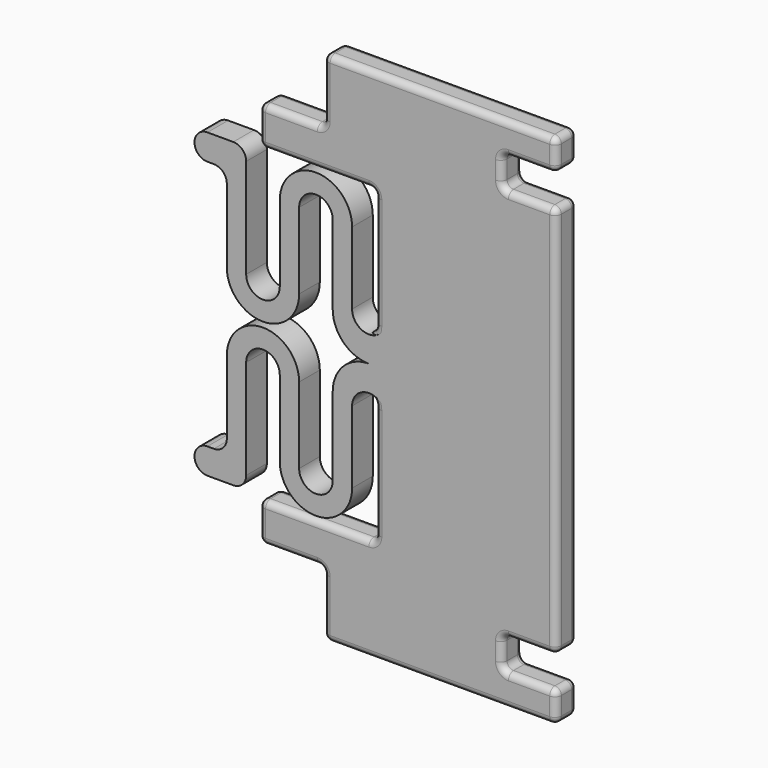
from build123d import *

# Parameters (mm, degrees)
F0_W          = 18
F0_H          = 2
F1_DEPTH      = 20
F2_W          = 4.2
F2_H          = 2.4
F3_DEPTH      = 2.001
F4_W          = 4
F4_H          = 12
F5_DEPTH      = 2.001
F6_W          = 5
F6_H          = 3
F7_DEPTH      = 2
F8_T1_DEPTH   = 2
F8_T3_DEPTH   = 2
F8_T5_DEPTH   = 7
F8_T7_DEPTH   = 7
F8_T9_DEPTH   = 7
F9_T1_DEPTH   = 2
F9_T3_DEPTH   = 18.75
F9_T5_DEPTH   = 1
F9_T7_DEPTH   = 4.5
F9_T9_DEPTH   = 3.15
F9_T11_DEPTH  = 17.7
F9_T13_DEPTH  = 5.5
F9_S17_W      = 0.5
F9_S17_H      = 0.5
F9_T18_DEPTH  = 0.5
F9_S23_W      = 0.5
F9_S23_H      = 0.5
F9_T24_DEPTH  = 0.5
F9_T27_DEPTH  = 1.4
F9_T29_DEPTH  = 3.2
F9_T31_DEPTH  = 8
F9_T33_DEPTH  = 4
F9_T35_DEPTH  = 4
F9_T37_DEPTH  = 8.6339745962
F9_S41_W      = 0.5
F9_S41_H      = 0.5
F9_T42_DEPTH  = 0.5
F9_S47_W      = 0.5
F9_S47_H      = 0.5
F9_T48_DEPTH  = 0.5
F9_S53_W      = 0.5
F9_S53_H      = 0.5
F9_T54_DEPTH  = 0.5
F9_S59_W      = 0.5
F9_S59_H      = 0.5
F9_T60_DEPTH  = 0.5
F9_S65_W      = 0.5
F9_S65_H      = 0.5
F9_T66_DEPTH  = 0.5
F9_S71_W      = 0.5
F9_S71_H      = 0.5
F9_T72_DEPTH  = 0.5
F9_S77_W      = 0.5
F9_S77_H      = 0.5
F9_T78_DEPTH  = 0.5
F9_S83_W      = 0.5
F9_S83_H      = 0.5
F9_T84_DEPTH  = 0.5
F9_S89_W      = 0.5
F9_S89_H      = 0.5
F9_T90_DEPTH  = 0.5
F9_S95_W      = 0.5
F9_S95_H      = 0.5
F9_T96_DEPTH  = 0.5
F9_T102_ANGLE = 131.6325091679
F9_S103_R     = 1.3
F9_T104_DEPTH = 3
F9_T108_ANGLE = 131.6325091679
F9_S109_R     = 1.3
F9_T110_DEPTH = 3
F9_T112_ANGLE = 90
F9_T114_ANGLE = 90
F9_T116_ANGLE = 90
F9_T118_ANGLE = 90
F9_T120_ANGLE = 90
F9_T122_ANGLE = 90
F9_T124_ANGLE = 90
F9_T126_ANGLE = 90


# Not quite as in the source:
# - a fillet or chamfer that OpenCascade refuses, or shapes differently, is made with other operations: its cross-section is extruded or revolved along the edge and cut away or added


with BuildPart() as f1:
    # F0 (on Top) → F1 (new body)
    with BuildSketch(Plane.XY):
        with Locations((-9, 1)):
            Rectangle(F0_W, F0_H)
    extrude(amount=F1_DEPTH)

    # F2 (on Front) → F3 (cut, through all)
    with BuildSketch(Plane.XZ):
        with Locations((-2.1, 16.4)):
            Rectangle(F2_W, F2_H)
    extrude(amount=-F3_DEPTH, mode=Mode.SUBTRACT)

    # F4 (on Front) → F5 (cut, through all)
    with BuildSketch(Plane.XZ):
        with Locations((-16, 6)):
            Rectangle(F4_W, F4_H)
    extrude(amount=-F5_DEPTH, mode=Mode.SUBTRACT)

    # F6 (on Front) → F7 (join)
    with BuildSketch(Plane.XZ):
        with BuildLine():
            Line((-24, 3), (-24, 11.7))
            Line((-24, 11.7), (-28, 11.7))
            Line((-28, 11.7), (-28, 9.7))
            Line((-28, 9.7), (-25.5, 9.7))
            Line((-25.5, 9.7), (-25.5, 3))
            ThreePointArc((-25.5, 3), (-22.7, 0.2), (-19.9, 3))
            Line((-19.9, 3), (-19.9, 8.9))
            ThreePointArc((-19.9, 8.9), (-18.6, 10.2), (-17.3, 8.9))
            Line((-17.3, 8.9), (-17.3, 2.8))
            ThreePointArc((-17.3, 2.8), (-16.4798989873, 0.8201010127), (-14.5, 0))
            Line((-14.5, 0), (-14, 0))
            Line((-14, 0), (-14, 2))
            Line((-14, 2), (-14.5, 2))
            ThreePointArc((-14.5, 2), (-15.4192388155, 2.3807611845), (-15.8, 3.3))
            Line((-15.8, 3.3), (-15.8, 8.9))
            ThreePointArc((-15.8, 8.9), (-18.6, 11.7), (-21.4, 8.9))
            Line((-21.4, 8.9), (-21.4, 3))
            ThreePointArc((-21.4, 3), (-22.7, 1.7), (-24, 3))
        make_face()
        with Locations((-20.5, 13.5)):
            Rectangle(F6_W, F6_H)
    extrude(amount=-F7_DEPTH)

    # F8: fillet of radius 1 on 5 edges, made by hand

    # F8_s2 → F8_t1 (join)
    with BuildSketch(Plane.XZ.offset(-2)):
        with BuildLine():
            ThreePointArc((-14, 2.8660254038), (-14.1339745962, 2.3660254038), (-14.5, 2))
            Line((-14.5, 2), (-14, 2))
            Line((-14, 2), (-14, 2.8660254038))
        make_face()
    extrude(amount=F8_T1_DEPTH)

    # F8_s4 → F8_t3 (join)
    with BuildSketch(Plane.XZ.offset(-2)):
        with BuildLine():
            ThreePointArc((-25.5, 8.7), (-25.7928932188, 9.4071067812), (-26.5, 9.7))
            Line((-26.5, 9.7), (-25.5, 9.7))
            Line((-25.5, 9.7), (-25.5, 8.7))
        make_face()
    extrude(amount=F8_T3_DEPTH)

    # F8_s6 → F8_t5 (cut)
    with BuildSketch(Plane.XZ.offset(-4.5)):
        with BuildLine():
            ThreePointArc((-25, 11.7), (-24.2928932188, 11.4071067812), (-24, 10.7))
            Line((-24, 10.7), (-24, 11.7))
            Line((-24, 11.7), (-25, 11.7))
        make_face()
    extrude(amount=F8_T5_DEPTH, mode=Mode.SUBTRACT)

    # F8_s8 → F8_t7 (cut)
    with BuildSketch(Plane.XZ.offset(-4.5)):
        with BuildLine():
            ThreePointArc((-27, 11.7), (-27.7071067812, 11.4071067812), (-28, 10.7))
            Line((-28, 10.7), (-28, 11.7))
            Line((-28, 11.7), (-27, 11.7))
        make_face()
    extrude(amount=F8_T7_DEPTH, mode=Mode.SUBTRACT)

    # F8_s10 → F8_t9 (cut)
    with BuildSketch(Plane.XZ.offset(-4.5)):
        with BuildLine():
            ThreePointArc((-28, 10.7), (-27.7071067812, 9.9928932188), (-27, 9.7))
            Line((-27, 9.7), (-28, 9.7))
            Line((-28, 9.7), (-28, 10.7))
        make_face()
    extrude(amount=F8_T9_DEPTH, mode=Mode.SUBTRACT)

    # F9: fillet of radius 0.5 on 32 edges, made by hand

    # F9_s2 → F9_t1 (join)
    with BuildSketch(Plane.XZ.offset(-2)):
        with BuildLine():
            ThreePointArc((-3.7, 15.2), (-4.0535533906, 15.3464466094), (-4.2, 15.7))
            Line((-4.2, 15.7), (-4.2, 15.2))
            Line((-4.2, 15.2), (-3.7, 15.2))
        make_face()
        with BuildLine():
            ThreePointArc((-4.2, 17.1), (-4.0535533906, 17.4535533906), (-3.7, 17.6))
            Line((-3.7, 17.6), (-4.2, 17.6))
            Line((-4.2, 17.6), (-4.2, 17.1))
        make_face()
        with BuildLine():
            ThreePointArc((-14.5, 12), (-14.1464466094, 11.8535533906), (-14, 11.5))
            Line((-14, 11.5), (-14, 12))
            Line((-14, 12), (-14.5, 12))
        make_face()
        with BuildLine():
            ThreePointArc((-18, 15.5), (-18.1464466094, 15.1464466094), (-18.5, 15))
            Line((-18.5, 15), (-18, 15))
            Line((-18, 15), (-18, 15.5))
        make_face()
    extrude(amount=F9_T1_DEPTH)

    # F9_s4 → F9_t3 (cut)
    with BuildSketch(Plane.YZ.offset(-19.25)):
        with BuildLine():
            ThreePointArc((0, 19.5), (0.1464466094, 19.8535533906), (0.5, 20))
            Line((0.5, 20), (0, 20))
            Line((0, 20), (0, 19.5))
        make_face()
        with BuildLine():
            ThreePointArc((2, 19.5), (1.8535533906, 19.8535533906), (1.5, 20))
            Line((1.5, 20), (2, 20))
            Line((2, 20), (2, 19.5))
        make_face()
    extrude(amount=F9_T3_DEPTH, mode=Mode.SUBTRACT)

    # F9_s6 → F9_t5 (cut)
    with BuildSketch(Plane.XZ.offset(-1.5)):
        with BuildLine():
            ThreePointArc((0, 19.5), (-0.1464466094, 19.8535533906), (-0.5, 20))
            Line((-0.5, 20), (0, 20))
            Line((0, 20), (0, 19.5))
        make_face()
    extrude(amount=F9_T5_DEPTH, mode=Mode.SUBTRACT)

    # F9_s8 → F9_t7 (cut)
    with BuildSketch(Plane.XZ.offset(-3.25)):
        with BuildLine():
            ThreePointArc((-17.5, 20), (-17.8535533906, 19.8535533906), (-18, 19.5))
            Line((-18, 19.5), (-18, 20))
            Line((-18, 20), (-17.5, 20))
        make_face()
        with BuildLine():
            ThreePointArc((-0.5, 17.6), (-0.1464466094, 17.7464466094), (0, 18.1))
            Line((0, 18.1), (0, 17.6))
            Line((0, 17.6), (-0.5, 17.6))
        make_face()
        with BuildLine():
            ThreePointArc((0, 14.7), (-0.1464466094, 15.0535533906), (-0.5, 15.2))
            Line((-0.5, 15.2), (0, 15.2))
            Line((0, 15.2), (0, 14.7))
        make_face()
        with BuildLine():
            ThreePointArc((-23, 12.5), (-22.8535533906, 12.1464466094), (-22.5, 12))
            Line((-22.5, 12), (-23, 12))
            Line((-23, 12), (-23, 12.5))
        make_face()
        with BuildLine():
            ThreePointArc((-22.5, 15), (-22.8535533906, 14.8535533906), (-23, 14.5))
            Line((-23, 14.5), (-23, 15))
            Line((-23, 15), (-22.5, 15))
        make_face()
    extrude(amount=F9_T7_DEPTH, mode=Mode.SUBTRACT)

    # F9_s10 → F9_t9 (cut)
    with BuildSketch(Plane.XY.offset(16.35)):
        with BuildLine():
            ThreePointArc((-0.5, 0), (-0.1464466094, 0.1464466094), (0, 0.5))
            Line((0, 0.5), (0, 0))
            Line((0, 0), (-0.5, 0))
        make_face()
        with BuildLine():
            ThreePointArc((-0.5, 2), (-0.1464466094, 1.8535533906), (0, 1.5))
            Line((0, 1.5), (0, 2))
            Line((0, 2), (-0.5, 2))
        make_face()
    extrude(amount=F9_T9_DEPTH, mode=Mode.SUBTRACT)

    # F9_s12 → F9_t11 (cut)
    with BuildSketch(Plane.XY.offset(-1.25)):
        with BuildLine():
            ThreePointArc((-0.5, 0), (-0.1464466094, 0.1464466094), (0, 0.5))
            Line((0, 0.5), (0, 0))
            Line((0, 0), (-0.5, 0))
        make_face()
        with BuildLine():
            ThreePointArc((0, 1.5), (-0.1464466094, 1.8535533906), (-0.5, 2))
            Line((-0.5, 2), (0, 2))
            Line((0, 2), (0, 1.5))
        make_face()
    extrude(amount=F9_T11_DEPTH, mode=Mode.SUBTRACT)

    # F9_s14 → F9_t13 (cut)
    with BuildSketch(Plane.XY.offset(10.75)):
        with BuildLine():
            ThreePointArc((-22.5, 0), (-22.8535533906, 0.1464466094), (-23, 0.5))
            Line((-23, 0.5), (-23, 0))
            Line((-23, 0), (-22.5, 0))
        make_face()
        with BuildLine():
            ThreePointArc((-22.5, 2), (-22.8535533906, 1.8535533906), (-23, 1.5))
            Line((-23, 1.5), (-23, 2))
            Line((-23, 2), (-22.5, 2))
        make_face()
    extrude(amount=F9_T13_DEPTH, mode=Mode.SUBTRACT)


with BuildPart() as f9_tool16:
    # F9_s17 → F9_t18 (new body)
    with BuildSketch(Plane.XZ.offset(-0.5)):
        with Locations((-0.25, 19.75)):
            Rectangle(F9_S17_W, F9_S17_H)
    extrude(amount=F9_T18_DEPTH)

    # F9_s19 → F9_t20 (revolve, cut)
    with BuildSketch(Plane(origin=(-0.5, 0.5, 19.5), x_dir=(-0.7071067812, 0, -0.7071067812), z_dir=(-0.7071067812, 0, 0.7071067812))):
        with BuildLine():
            ThreePointArc((0, -0.5), (0.5, 0), (0, 0.5))
            Line((0, 0.5), (0, -0.5))
        make_face()
    revolve(axis=Axis((-0.5, 0.5, 19.5), (0, -1, 0)), mode=Mode.SUBTRACT)


with BuildPart() as f1_1:
    add(f1.part)

    # F9_t15: cut F9_tool16
    add(f9_tool16.part, mode=Mode.SUBTRACT)


with BuildPart() as f9_tool22:
    # F9_s23 → F9_t24 (new body)
    with BuildSketch(Plane.YZ.offset(-0.5)):
        with Locations((1.75, 19.75)):
            Rectangle(F9_S23_W, F9_S23_H)
    extrude(amount=F9_T24_DEPTH)

    # F9_s25 → F9_t26 (revolve, cut)
    with BuildSketch(Plane(origin=(-0.5, 1.5, 19.5), x_dir=(0, -0.7071067812, -0.7071067812), z_dir=(0, -0.7071067812, 0.7071067812))):
        with BuildLine():
            ThreePointArc((0, -0.5), (0.5, 0), (0, 0.5))
            Line((0, 0.5), (0, -0.5))
        make_face()
    revolve(axis=Axis((-0.5, 1.5, 19.5), (1, 0, 0)), mode=Mode.SUBTRACT)


with BuildPart() as f1_2:
    add(f1_1.part)

    # F9_t21: cut F9_tool22
    add(f9_tool22.part, mode=Mode.SUBTRACT)

    # F9_s28 → F9_t27 (cut)
    with BuildSketch(Plane.XY.offset(15.7)):
        with BuildLine():
            ThreePointArc((-4.7, 0), (-4.3464466094, 0.1464466094), (-4.2, 0.5))
            Line((-4.2, 0.5), (-4.2, 0))
            Line((-4.2, 0), (-4.7, 0))
        make_face()
        with BuildLine():
            ThreePointArc((-4.2, 1.5), (-4.3464466094, 1.8535533906), (-4.7, 2))
            Line((-4.7, 2), (-4.2, 2))
            Line((-4.2, 2), (-4.2, 1.5))
        make_face()
    extrude(amount=F9_T27_DEPTH, mode=Mode.SUBTRACT)

    # F9_s30 → F9_t29 (cut)
    with BuildSketch(Plane.YZ.offset(-3.7)):
        with BuildLine():
            ThreePointArc((0, 14.7), (0.1464466094, 15.0535533906), (0.5, 15.2))
            Line((0.5, 15.2), (0, 15.2))
            Line((0, 15.2), (0, 14.7))
        make_face()
        with BuildLine():
            ThreePointArc((1.5, 15.2), (1.8535533906, 15.0535533906), (2, 14.7))
            Line((2, 14.7), (2, 15.2))
            Line((2, 15.2), (1.5, 15.2))
        make_face()
        with BuildLine():
            ThreePointArc((0, 18.1), (0.1464466094, 17.7464466094), (0.5, 17.6))
            Line((0.5, 17.6), (0, 17.6))
            Line((0, 17.6), (0, 18.1))
        make_face()
        with BuildLine():
            ThreePointArc((1.5, 17.6), (1.8535533906, 17.7464466094), (2, 18.1))
            Line((2, 18.1), (2, 17.6))
            Line((2, 17.6), (1.5, 17.6))
        make_face()
    extrude(amount=F9_T29_DEPTH, mode=Mode.SUBTRACT)

    # F9_s32 → F9_t31 (cut)
    with BuildSketch(Plane.YZ.offset(-22.5)):
        with BuildLine():
            ThreePointArc((1.5, 12), (1.8535533906, 12.1464466094), (2, 12.5))
            Line((2, 12.5), (2, 12))
            Line((2, 12), (1.5, 12))
        make_face()
        with BuildLine():
            ThreePointArc((0, 12.5), (0.1464466094, 12.1464466094), (0.5, 12))
            Line((0.5, 12), (0, 12))
            Line((0, 12), (0, 12.5))
        make_face()
    extrude(amount=F9_T31_DEPTH, mode=Mode.SUBTRACT)

    # F9_s34 → F9_t33 (cut)
    with BuildSketch(Plane.XY.offset(15.5)):
        with BuildLine():
            ThreePointArc((-17.5, 0), (-17.8535533906, 0.1464466094), (-18, 0.5))
            Line((-18, 0.5), (-18, 0))
            Line((-18, 0), (-17.5, 0))
        make_face()
        with BuildLine():
            ThreePointArc((-18, 1.5), (-17.8535533906, 1.8535533906), (-17.5, 2))
            Line((-17.5, 2), (-18, 2))
            Line((-18, 2), (-18, 1.5))
        make_face()
    extrude(amount=F9_T33_DEPTH, mode=Mode.SUBTRACT)

    # F9_s36 → F9_t35 (cut)
    with BuildSketch(Plane.YZ.offset(-22.5)):
        with BuildLine():
            ThreePointArc((0, 14.5), (0.1464466094, 14.8535533906), (0.5, 15))
            Line((0.5, 15), (0, 15))
            Line((0, 15), (0, 14.5))
        make_face()
        with BuildLine():
            ThreePointArc((1.5, 15), (1.8535533906, 14.8535533906), (2, 14.5))
            Line((2, 14.5), (2, 15))
            Line((2, 15), (1.5, 15))
        make_face()
    extrude(amount=F9_T35_DEPTH, mode=Mode.SUBTRACT)

    # F9_s38 → F9_t37 (cut)
    with BuildSketch(Plane.XY.offset(2.8660254038)):
        with BuildLine():
            ThreePointArc((-13.5, 0), (-13.8535533906, 0.1464466094), (-14, 0.5))
            Line((-14, 0.5), (-14, 0))
            Line((-14, 0), (-13.5, 0))
        make_face()
        with BuildLine():
            ThreePointArc((-14, 1.5), (-13.8535533906, 1.8535533906), (-13.5, 2))
            Line((-13.5, 2), (-14, 2))
            Line((-14, 2), (-14, 1.5))
        make_face()
    extrude(amount=F9_T37_DEPTH, mode=Mode.SUBTRACT)


with BuildPart() as f9_tool40:
    # F9_s41 → F9_t42 (new body)
    with BuildSketch(Plane.XY.offset(18.1)):
        with Locations((-0.25, 1.75)):
            Rectangle(F9_S41_W, F9_S41_H)
    extrude(amount=-F9_T42_DEPTH)

    # F9_s43 → F9_t44 (revolve, cut)
    with BuildSketch(Plane(origin=(-0.5, 1.5, 18.1), x_dir=(-0.7071067812, -0.7071067812, 0), z_dir=(0.7071067812, -0.7071067812, 0))):
        with BuildLine():
            ThreePointArc((0, -0.5), (0.5, 0), (0, 0.5))
            Line((0, 0.5), (0, -0.5))
        make_face()
    revolve(axis=Axis((-0.5, 1.5, 18.1), (0, 0, -1)), mode=Mode.SUBTRACT)


with BuildPart() as f1_3:
    add(f1_2.part)

    # F9_t39: cut F9_tool40
    add(f9_tool40.part, mode=Mode.SUBTRACT)


with BuildPart() as f9_tool46:
    # F9_s47 → F9_t48 (new body)
    with BuildSketch(Plane.XZ.offset(-0.5)):
        with Locations((-0.25, 17.85)):
            Rectangle(F9_S47_W, F9_S47_H)
    extrude(amount=F9_T48_DEPTH)

    # F9_s49 → F9_t50 (revolve, cut)
    with BuildSketch(Plane(origin=(-0.5, 0.5, 18.1), x_dir=(-0.7071067812, 0, 0.7071067812), z_dir=(0.7071067812, 0, 0.7071067812))):
        with BuildLine():
            ThreePointArc((0, -0.5), (0.5, 0), (0, 0.5))
            Line((0, 0.5), (0, -0.5))
        make_face()
    revolve(axis=Axis((-0.5, 0.5, 18.1), (0, -1, 0)), mode=Mode.SUBTRACT)


with BuildPart() as f1_4:
    add(f1_3.part)

    # F9_t45: cut F9_tool46
    add(f9_tool46.part, mode=Mode.SUBTRACT)


with BuildPart() as f9_tool52:
    # F9_s53 → F9_t54 (new body)
    with BuildSketch(Plane.XY.offset(14.5)):
        with Locations((-22.75, 1.75)):
            Rectangle(F9_S53_W, F9_S53_H)
    extrude(amount=F9_T54_DEPTH)

    # F9_s55 → F9_t56 (revolve, cut)
    with BuildSketch(Plane(origin=(-22.5, 1.5, 14.5), x_dir=(0.7071067812, -0.7071067812, 0), z_dir=(-0.7071067812, -0.7071067812, 0))):
        with BuildLine():
            ThreePointArc((0, -0.5), (0.5, 0), (0, 0.5))
            Line((0, 0.5), (0, -0.5))
        make_face()
    revolve(axis=Axis((-22.5, 1.5, 14.5), (0, 0, 1)), mode=Mode.SUBTRACT)


with BuildPart() as f1_5:
    add(f1_4.part)

    # F9_t51: cut F9_tool52
    add(f9_tool52.part, mode=Mode.SUBTRACT)


with BuildPart() as f9_tool58:
    # F9_s59 → F9_t60 (new body)
    with BuildSketch(Plane.XZ.offset(-0.5)):
        with Locations((-22.75, 14.75)):
            Rectangle(F9_S59_W, F9_S59_H)
    extrude(amount=F9_T60_DEPTH)

    # F9_s61 → F9_t62 (revolve, cut)
    with BuildSketch(Plane(origin=(-22.5, 0.5, 14.5), x_dir=(0.7071067812, 0, -0.7071067812), z_dir=(-0.7071067812, 0, -0.7071067812))):
        with BuildLine():
            ThreePointArc((0, -0.5), (0.5, 0), (0, 0.5))
            Line((0, 0.5), (0, -0.5))
        make_face()
    revolve(axis=Axis((-22.5, 0.5, 14.5), (0, -1, 0)), mode=Mode.SUBTRACT)


with BuildPart() as f1_6:
    add(f1_5.part)

    # F9_t57: cut F9_tool58
    add(f9_tool58.part, mode=Mode.SUBTRACT)


with BuildPart() as f9_tool64:
    # F9_s65 → F9_t66 (new body)
    with BuildSketch(Plane.YZ.offset(-17.5)):
        with Locations((1.75, 19.75)):
            Rectangle(F9_S65_W, F9_S65_H)
    extrude(amount=-F9_T66_DEPTH)

    # F9_s67 → F9_t68 (revolve, cut)
    with BuildSketch(Plane(origin=(-17.5, 1.5, 19.5), x_dir=(0, -0.7071067812, -0.7071067812), z_dir=(0, 0.7071067812, -0.7071067812))):
        with BuildLine():
            ThreePointArc((0, -0.5), (0.5, 0), (0, 0.5))
            Line((0, 0.5), (0, -0.5))
        make_face()
    revolve(axis=Axis((-17.5, 1.5, 19.5), (-1, 0, 0)), mode=Mode.SUBTRACT)


with BuildPart() as f1_7:
    add(f1_6.part)

    # F9_t63: cut F9_tool64
    add(f9_tool64.part, mode=Mode.SUBTRACT)


with BuildPart() as f9_tool70:
    # F9_s71 → F9_t72 (new body)
    with BuildSketch(Plane.XZ.offset(-0.5)):
        with Locations((-17.75, 19.75)):
            Rectangle(F9_S71_W, F9_S71_H)
    extrude(amount=F9_T72_DEPTH)

    # F9_s73 → F9_t74 (revolve, cut)
    with BuildSketch(Plane(origin=(-17.5, 0.5, 19.5), x_dir=(0.7071067812, 0, -0.7071067812), z_dir=(-0.7071067812, 0, -0.7071067812))):
        with BuildLine():
            ThreePointArc((0, -0.5), (0.5, 0), (0, 0.5))
            Line((0, 0.5), (0, -0.5))
        make_face()
    revolve(axis=Axis((-17.5, 0.5, 19.5), (0, -1, 0)), mode=Mode.SUBTRACT)


with BuildPart() as f1_8:
    add(f1_7.part)

    # F9_t69: cut F9_tool70
    add(f9_tool70.part, mode=Mode.SUBTRACT)


with BuildPart() as f9_tool76:
    # F9_s77 → F9_t78 (new body)
    with BuildSketch(Plane.XZ.offset(-0.5)):
        with Locations((-22.75, 12.25)):
            Rectangle(F9_S77_W, F9_S77_H)
    extrude(amount=F9_T78_DEPTH)

    # F9_s79 → F9_t80 (revolve, cut)
    with BuildSketch(Plane(origin=(-22.5, 0.5, 12.5), x_dir=(0.7071067812, 0, 0.7071067812), z_dir=(0.7071067812, 0, -0.7071067812))):
        with BuildLine():
            ThreePointArc((0, -0.5), (0.5, 0), (0, 0.5))
            Line((0, 0.5), (0, -0.5))
        make_face()
    revolve(axis=Axis((-22.5, 0.5, 12.5), (0, -1, 0)), mode=Mode.SUBTRACT)


with BuildPart() as f1_9:
    add(f1_8.part)

    # F9_t75: cut F9_tool76
    add(f9_tool76.part, mode=Mode.SUBTRACT)


with BuildPart() as f9_tool82:
    # F9_s83 → F9_t84 (new body)
    with BuildSketch(Plane.XY.offset(12.5)):
        with Locations((-22.75, 1.75)):
            Rectangle(F9_S83_W, F9_S83_H)
    extrude(amount=-F9_T84_DEPTH)

    # F9_s85 → F9_t86 (revolve, cut)
    with BuildSketch(Plane(origin=(-22.5, 1.5, 12.5), x_dir=(0.7071067812, -0.7071067812, 0), z_dir=(0.7071067812, 0.7071067812, 0))):
        with BuildLine():
            ThreePointArc((0, -0.5), (0.5, 0), (0, 0.5))
            Line((0, 0.5), (0, -0.5))
        make_face()
    revolve(axis=Axis((-22.5, 1.5, 12.5), (0, 0, -1)), mode=Mode.SUBTRACT)


with BuildPart() as f1_10:
    add(f1_9.part)

    # F9_t81: cut F9_tool82
    add(f9_tool82.part, mode=Mode.SUBTRACT)


with BuildPart() as f9_tool88:
    # F9_s89 → F9_t90 (new body)
    with BuildSketch(Plane.XY.offset(14.7)):
        with Locations((-0.25, 1.75)):
            Rectangle(F9_S89_W, F9_S89_H)
    extrude(amount=F9_T90_DEPTH)

    # F9_s91 → F9_t92 (revolve, cut)
    with BuildSketch(Plane(origin=(-0.5, 1.5, 14.7), x_dir=(-0.7071067812, -0.7071067812, 0), z_dir=(-0.7071067812, 0.7071067812, 0))):
        with BuildLine():
            ThreePointArc((0, -0.5), (0.5, 0), (0, 0.5))
            Line((0, 0.5), (0, -0.5))
        make_face()
    revolve(axis=Axis((-0.5, 1.5, 14.7), (0, 0, 1)), mode=Mode.SUBTRACT)


with BuildPart() as f1_11:
    add(f1_10.part)

    # F9_t87: cut F9_tool88
    add(f9_tool88.part, mode=Mode.SUBTRACT)


with BuildPart() as f9_tool94:
    # F9_s95 → F9_t96 (new body)
    with BuildSketch(Plane.XZ.offset(-0.5)):
        with Locations((-0.25, 14.95)):
            Rectangle(F9_S95_W, F9_S95_H)
    extrude(amount=F9_T96_DEPTH)

    # F9_s97 → F9_t98 (revolve, cut)
    with BuildSketch(Plane(origin=(-0.5, 0.5, 14.7), x_dir=(-0.7071067812, 0, -0.7071067812), z_dir=(-0.7071067812, 0, 0.7071067812))):
        with BuildLine():
            ThreePointArc((0, -0.5), (0.5, 0), (0, 0.5))
            Line((0, 0.5), (0, -0.5))
        make_face()
    revolve(axis=Axis((-0.5, 0.5, 14.7), (0, -1, 0)), mode=Mode.SUBTRACT)


with BuildPart() as f1_12:
    add(f1_11.part)

    # F9_t93: cut F9_tool94
    add(f9_tool94.part, mode=Mode.SUBTRACT)


with BuildPart() as f9_tool100:
    # F9_s101 → F9_t102 (revolve)
    with BuildSketch(Plane.XY.offset(2.8660254038)):
        with BuildLine():
            ThreePointArc((-14, 1.5), (-13.8535533906, 1.8535533906), (-13.5, 2))
            Line((-13.5, 2), (-14, 2))
            Line((-14, 2), (-14, 1.5))
        make_face()
    revolve(axis=Axis((-15, 2, 2.8660254038), (0, 1, 0)), revolution_arc=F9_T102_ANGLE)

    # F9_s103 → F9_t104 (intersect, symmetric)
    with BuildSketch(Plane.XZ.offset(-1.8)):
        with Locations((-14.5, 3.3)):
            Circle(F9_S103_R)
    extrude(amount=F9_T104_DEPTH, both=True, mode=Mode.INTERSECT)


with BuildPart() as f1_13:
    add(f1_12.part)

    # F9_t99: cut F9_tool100
    add(f9_tool100.part, mode=Mode.SUBTRACT)


with BuildPart() as f9_tool106:
    # F9_s107 → F9_t108 (revolve)
    with BuildSketch(Plane.XY.offset(2.8660254038)):
        with BuildLine():
            ThreePointArc((-13.5, 0), (-13.8535533906, 0.1464466094), (-14, 0.5))
            Line((-14, 0.5), (-14, 0))
            Line((-14, 0), (-13.5, 0))
        make_face()
    revolve(axis=Axis((-15, 0, 2.8660254038), (0, 1, 0)), revolution_arc=F9_T108_ANGLE)

    # F9_s109 → F9_t110 (intersect, symmetric)
    with BuildSketch(Plane.XZ.offset(-0.4)):
        with Locations((-14.5, 3.3)):
            Circle(F9_S109_R)
    extrude(amount=F9_T110_DEPTH, both=True, mode=Mode.INTERSECT)


with BuildPart() as f1_14:
    add(f1_13.part)

    # F9_t105: cut F9_tool106
    add(f9_tool106.part, mode=Mode.SUBTRACT)

    # F9_s111 → F9_t112 (revolve, cut)
    with BuildSketch(Plane.YZ.offset(-14.5)):
        with BuildLine():
            ThreePointArc((1.5, 12), (1.8535533906, 12.1464466094), (2, 12.5))
            Line((2, 12.5), (2, 12))
            Line((2, 12), (1.5, 12))
        make_face()
    revolve(axis=Axis((-14.5, 2, 11.5), (0, 1, 0)), revolution_arc=F9_T112_ANGLE, mode=Mode.SUBTRACT)

    # F9_s113 → F9_t114 (revolve, cut)
    with BuildSketch(Plane.XY.offset(17.1)):
        with BuildLine():
            ThreePointArc((-4.2, 1.5), (-4.3464466094, 1.8535533906), (-4.7, 2))
            Line((-4.7, 2), (-4.2, 2))
            Line((-4.2, 2), (-4.2, 1.5))
        make_face()
    revolve(axis=Axis((-3.7, 2, 17.1), (0, 1, 0)), revolution_arc=F9_T114_ANGLE, mode=Mode.SUBTRACT)

    # F9_s115 → F9_t116 (revolve, cut)
    with BuildSketch(Plane.YZ.offset(-14.5)):
        with BuildLine():
            ThreePointArc((0, 12.5), (0.1464466094, 12.1464466094), (0.5, 12))
            Line((0.5, 12), (0, 12))
            Line((0, 12), (0, 12.5))
        make_face()
    revolve(axis=Axis((-14.5, 0, 11.5), (0, 1, 0)), revolution_arc=F9_T116_ANGLE, mode=Mode.SUBTRACT)

    # F9_s117 → F9_t118 (revolve, cut)
    with BuildSketch(Plane.XY.offset(17.1)):
        with BuildLine():
            ThreePointArc((-4.7, 0), (-4.3464466094, 0.1464466094), (-4.2, 0.5))
            Line((-4.2, 0.5), (-4.2, 0))
            Line((-4.2, 0), (-4.7, 0))
        make_face()
    revolve(axis=Axis((-3.7, 0, 17.1), (0, 1, 0)), revolution_arc=F9_T118_ANGLE, mode=Mode.SUBTRACT)

    # F9_s119 → F9_t120 (revolve, cut)
    with BuildSketch(Plane.XY.offset(15.5)):
        with BuildLine():
            ThreePointArc((-18, 1.5), (-17.8535533906, 1.8535533906), (-17.5, 2))
            Line((-17.5, 2), (-18, 2))
            Line((-18, 2), (-18, 1.5))
        make_face()
    revolve(axis=Axis((-18.5, 2, 15.5), (0, 1, 0)), revolution_arc=F9_T120_ANGLE, mode=Mode.SUBTRACT)

    # F9_s121 → F9_t122 (revolve, cut)
    with BuildSketch(Plane.XY.offset(15.5)):
        with BuildLine():
            ThreePointArc((-17.5, 0), (-17.8535533906, 0.1464466094), (-18, 0.5))
            Line((-18, 0.5), (-18, 0))
            Line((-18, 0), (-17.5, 0))
        make_face()
    revolve(axis=Axis((-18.5, 0, 15.5), (0, 1, 0)), revolution_arc=F9_T122_ANGLE, mode=Mode.SUBTRACT)

    # F9_s123 → F9_t124 (revolve, cut)
    with BuildSketch(Plane.YZ.offset(-3.7)):
        with BuildLine():
            ThreePointArc((1.5, 15.2), (1.8535533906, 15.0535533906), (2, 14.7))
            Line((2, 14.7), (2, 15.2))
            Line((2, 15.2), (1.5, 15.2))
        make_face()
    revolve(axis=Axis((-3.7, 2, 15.7), (0, 1, 0)), revolution_arc=F9_T124_ANGLE, mode=Mode.SUBTRACT)

    # F9_s125 → F9_t126 (revolve, cut)
    with BuildSketch(Plane.YZ.offset(-3.7)):
        with BuildLine():
            ThreePointArc((0, 14.7), (0.1464466094, 15.0535533906), (0.5, 15.2))
            Line((0.5, 15.2), (0, 15.2))
            Line((0, 15.2), (0, 14.7))
        make_face()
    revolve(axis=Axis((-3.7, 0, 15.7), (0, 1, 0)), revolution_arc=F9_T126_ANGLE, mode=Mode.SUBTRACT)

    # F10: F1 across plane


with BuildPart() as f1_15:
    add(f1_14.part)
    add(f1_14.part.mirror(Plane.XY))


solid = f1_15.part
